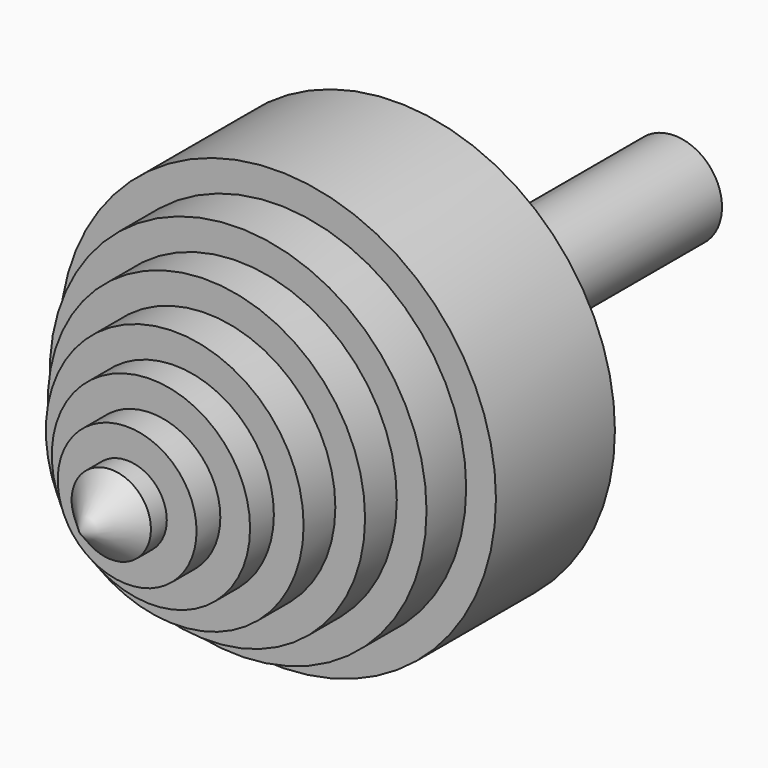
from build123d import *

# Parameters (mm, degrees)
F0_R      = 22
F0_R_2    = 19
F0_R_3    = 16
F0_R_4    = 13
F0_R_5    = 10
F0_R_6    = 7
F0_R_7    = 4
F1_DEPTH  = 15
F2_DEPTH  = 20
F3_DEPTH  = 24
F4_DEPTH  = 28
F5_DEPTH  = 31
F6_DEPTH  = 34
F7_DEPTH  = 40
F8_SIZE   = 4
F9_R      = 17.5
F10_DEPTH = 3
F11_R     = 11.5
F12_DEPTH = 2
F13_R     = 4.8
F14_DEPTH = 30
F15_R     = 1.5
F16_DEPTH = 12.5


# Not quite as in the source:
# - a feature names something its author has since deleted; it is built from what else it names


with BuildPart() as f1:
    # F0 (on Front) → F1 (new body)
    with BuildSketch(Plane.XZ):
        Circle(F0_R)
        Circle(F0_R_2, mode=Mode.SUBTRACT)
        Circle(F0_R_2)
        Circle(F0_R_3, mode=Mode.SUBTRACT)
        Circle(F0_R_3)
        Circle(F0_R_4, mode=Mode.SUBTRACT)
        Circle(F0_R_4)
        Circle(F0_R_5, mode=Mode.SUBTRACT)
        Circle(F0_R_5)
        Circle(F0_R_6, mode=Mode.SUBTRACT)
        Circle(F0_R_6)
        Circle(F0_R_7, mode=Mode.SUBTRACT)
        Circle(F0_R_7)
    extrude(amount=F1_DEPTH)

    # F0 (on Front) → F2 (join)
    with BuildSketch(Plane.XZ):
        Circle(F0_R_2)
        Circle(F0_R_3, mode=Mode.SUBTRACT)
        Circle(F0_R_3)
        Circle(F0_R_4, mode=Mode.SUBTRACT)
        Circle(F0_R_4)
        Circle(F0_R_5, mode=Mode.SUBTRACT)
        Circle(F0_R_5)
        Circle(F0_R_6, mode=Mode.SUBTRACT)
        Circle(F0_R_6)
        Circle(F0_R_7, mode=Mode.SUBTRACT)
        Circle(F0_R_7)
    extrude(amount=F2_DEPTH)

    # F0 (on Front) → F3 (join)
    with BuildSketch(Plane.XZ):
        Circle(F0_R_3)
        Circle(F0_R_4, mode=Mode.SUBTRACT)
        Circle(F0_R_4)
        Circle(F0_R_5, mode=Mode.SUBTRACT)
        Circle(F0_R_5)
        Circle(F0_R_6, mode=Mode.SUBTRACT)
        Circle(F0_R_6)
        Circle(F0_R_7, mode=Mode.SUBTRACT)
        Circle(F0_R_7)
    extrude(amount=F3_DEPTH)

    # F0 (on Front) → F4 (join)
    with BuildSketch(Plane.XZ):
        Circle(F0_R_4)
        Circle(F0_R_5, mode=Mode.SUBTRACT)
        Circle(F0_R_5)
        Circle(F0_R_6, mode=Mode.SUBTRACT)
        Circle(F0_R_6)
        Circle(F0_R_7, mode=Mode.SUBTRACT)
        Circle(F0_R_7)
    extrude(amount=F4_DEPTH)

    # F0 (on Front) → F5 (join)
    with BuildSketch(Plane.XZ):
        Circle(F0_R_5)
        Circle(F0_R_6, mode=Mode.SUBTRACT)
        Circle(F0_R_6)
        Circle(F0_R_7, mode=Mode.SUBTRACT)
        Circle(F0_R_7)
    extrude(amount=F5_DEPTH)

    # F0 (on Front) → F6 (join)
    with BuildSketch(Plane.XZ):
        Circle(F0_R_6)
        Circle(F0_R_7, mode=Mode.SUBTRACT)
        Circle(F0_R_7)
    extrude(amount=F6_DEPTH)

    # F0 (on Front) → F7 (join)
    with BuildSketch(Plane.XZ):
        Circle(F0_R_7)
    extrude(amount=F7_DEPTH)

    # F8
    f8_edges = [f1.edges().sort_by_distance(p)[0] for p in [
        (-4, -40, 0),
    ]]
    chamfer(f8_edges, length=F8_SIZE)

    # F9 (on face) → F10 (join)
    with BuildSketch(Plane(origin=(0, 0, 0), x_dir=(-1, 0, 0), z_dir=(0, 1, 0))):
        Circle(F9_R)
    extrude(amount=F10_DEPTH)

    # F11 (on face) → F12 (join)
    with BuildSketch(Plane(origin=(0, 3, 0), x_dir=(-1, 0, 0), z_dir=(0, 1, 0))):
        Circle(F11_R)
    extrude(amount=F12_DEPTH)

    # F13 (on face) → F14 (join)
    with BuildSketch(Plane(origin=(0, 5, 0), x_dir=(-1, 0, 0), z_dir=(0, 1, 0))):
        Circle(F13_R)
    extrude(amount=F14_DEPTH)

    # F15 (on Top) → F16 (cut, symmetric)
    with BuildSketch(Plane.XY):
        with Locations((0, 15)):
            Circle(F15_R)
    extrude(amount=F16_DEPTH, both=True, mode=Mode.SUBTRACT)


solid = f1.part
